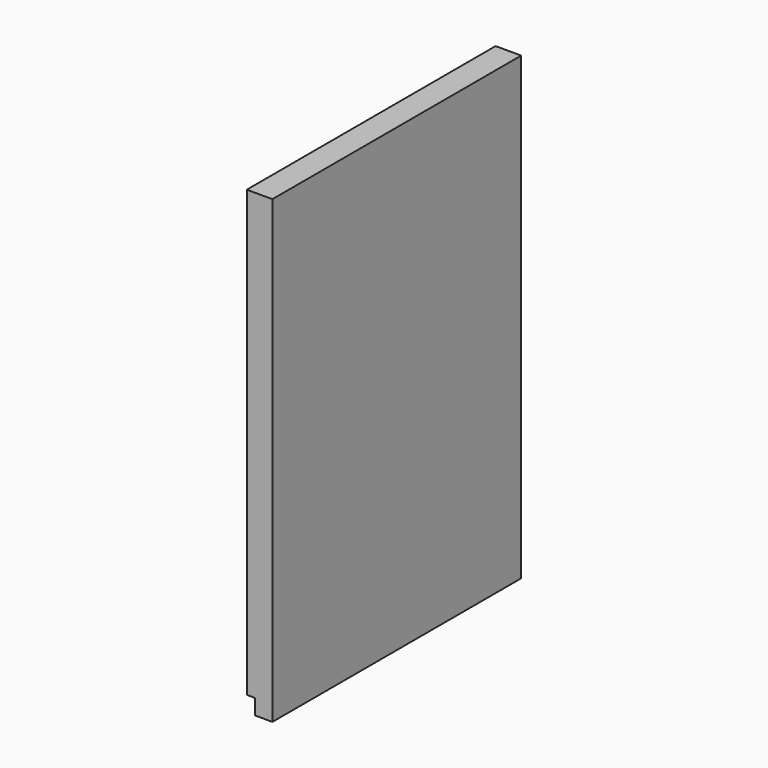
from build123d import *

# Parameters (mm, degrees)
F2_DEPTH = 330


# Not quite as in the source:
# - a feature of the source that left no trace in its solid (it failed there, or was rolled back) is left out


with BuildPart() as f2:
    # F0 (on Front) → F2 (new body)
    with BuildSketch(Plane.XZ):
        Polygon((-166.6411012411, 147.3953723907), (-166.6411012411, 163.9132797718), (-193.8388049603, 163.9132797718), (-193.8388049603, -308.0049455166), (-185.2051019669, -308.0049455166), (-185.2051019669, -324.4089782238), (-166.6411012411, -324.4089782238), align=None)
    extrude(amount=F2_DEPTH)


solid = f2.part
